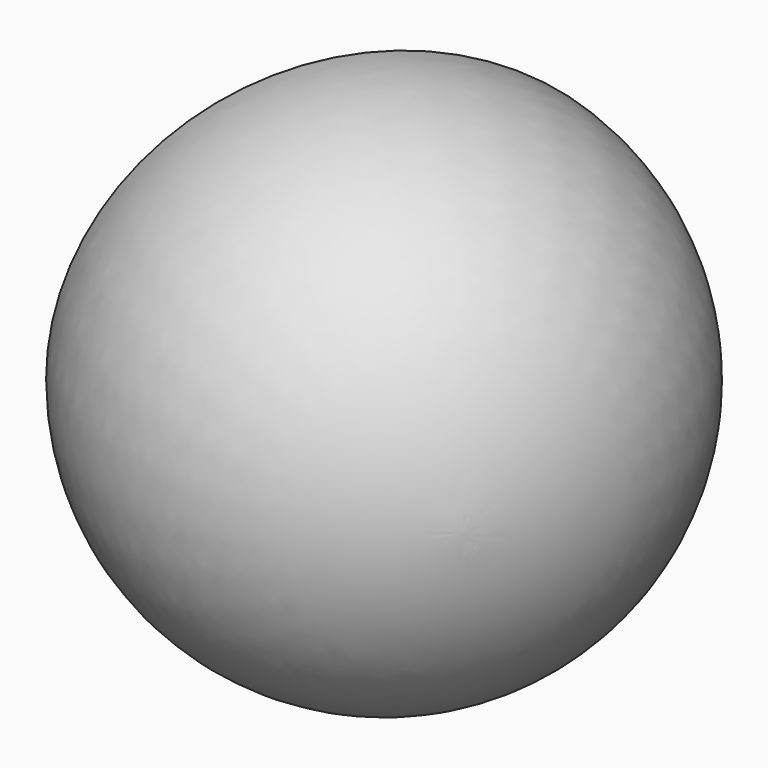
from build123d import *

# Parameters (mm, degrees)
F2_R     = 3.9307003836
F3_DEPTH = 3


# Not quite as in the source:
# - a fillet or chamfer that OpenCascade refuses, or shapes differently, is made with other operations: its cross-section is extruded or revolved along the edge and cut away or added


with BuildPart() as f1:
    # F0 (on Top) → F1 (revolve)
    with BuildSketch(Plane.XY):
        with BuildLine():
            Line((0, 0), (21.9969083539, 0))
            ThreePointArc((21.9969083539, 0), (10.998454177, 11.1844063915), (0, 0))
        make_face()
    revolve(axis=Axis((10.998454177, 0, 0), (-1, 0, 0)))

    # F2 (on Right) → F3 (join)
    with BuildSketch(Plane.YZ):
        Circle(F2_R)
    extrude(amount=F3_DEPTH)

    # F4: fillet of radius 2 on 1 edges, made by hand

    # F4_s1 → F4_t2 (revolve, cut)
    with BuildSketch(Plane.XY):
        with BuildLine():
            ThreePointArc((0.6560520708, 3.9307003833), (0.1713535254, 3.2595212556), (0, 2.449550842))
            Line((0, 2.449550842), (-0.04, 2.449550842))
            Line((-0.04, 2.449550842), (-0.04, 3.9307003836))
            Line((-0.04, 3.9307003836), (0, 3.9707003836))
            ThreePointArc((0, 3.9707003836), (0.3280260354, 3.9707003836), (0.6291731123, 3.9603233741))
            Line((0.6291731123, 3.9603233741), (0.6560520708, 3.9307003833))
        make_face()
    revolve(axis=Axis((0, 0, 0), (1, 0, 0)), mode=Mode.SUBTRACT)

    # F5 (on Top) → F6 (revolve)
    with BuildSketch(Plane.XY):
        with BuildLine():
            Line((8.5283361841, 1.7954872455), (1.753479708, -7.604626473))
            ThreePointArc((1.753479708, -7.604626473), (11.1456233489, -12.1186993884), (20.5377669899, -7.604626473))
            Line((20.5377669899, -7.604626473), (8.5283361841, 1.7954872455))
        make_face()
    revolve(axis=Axis((14.533051587, -2.9045696137, 0), (0.7874595304, -0.6163663586, 0)))


solid = f1.part
